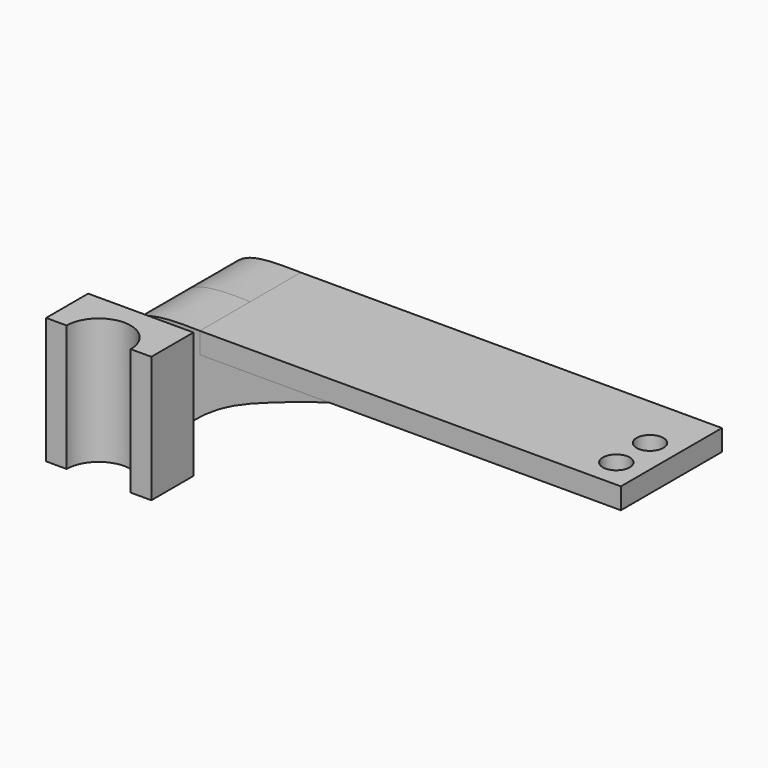
from build123d import *

# Parameters (mm, degrees)
F1_DEPTH      = 19.05
F2_DEPTH      = 19.05
F0_W          = 19.05
F0_H          = 19.05
F3_DEPTH      = 25.4
F3_DEPTH_BACK = 19.05
F4_W          = 31.75
F4_H          = 38.1
F4_W_2        = 19.05
F4_H_2        = 19.05
F5_DEPTH      = 15.875
F7_D          = 19.304
F9_D          = 8.128


with BuildPart() as f1:
    # F0 (on Front) → F1 (new body, symmetric)
    with BuildSketch(Plane.XZ):
        Polygon((73.453836826, -1.6650080707), (-53.546163174, -1.6650080707), (-53.546163174, -8.0150080707), (-14.6733894944, -8.0150080707), (73.453836826, -8.0150080707), align=None)
    extrude(amount=F1_DEPTH, both=True)

    # F9 (through all)
    with Locations(Plane(origin=(0, 0, -8.0150080707), x_dir=(1, 0, 0), z_dir=(0, 0, -1))):
        with Locations((64.970236826, 10.16), (64.970236826, -2.54)):
            Hole(F9_D / 2)


with BuildPart() as f2:
    # F0 (on Front) → F2 (new body, symmetric)
    with BuildSketch(Plane.XZ):
        with BuildLine():
            add(Edge.make_bspline(
                [(-75.771163174, -8.0150080707), (-74.1607508996, -6.1029628681), (-70.2003043439, -1.40071801), (-59.7481949502, -1.5665859823), (-53.546163174, -1.6650080707)],
                knots=[0, 0, 0, 0, 0.4066239127, 1, 1, 1, 1], degree=3))
            Line((-75.771163174, -8.0150080707), (-56.721163174, -8.0150080707))
            Line((-56.721163174, -8.0150080707), (-56.721163174, -27.0650080707))
            add(Edge.make_bspline(
                [(-56.721163174, -27.0650080707), (-53.3356832439, -24.3351180324), (-44.8730943092, -17.5112887062), (-25.9976593517, -11.5759185238), (-14.6733894944, -8.0150080707)],
                knots=[0, 0, 0, 0, 0.4000525083, 1, 1, 1, 1], degree=3))
            Line((-14.6733894944, -8.0150080707), (-53.546163174, -8.0150080707))
            Line((-53.546163174, -8.0150080707), (-53.546163174, -1.6650080707))
        make_face()
    extrude(amount=F2_DEPTH, both=True)


with BuildPart() as f3:
    # F0 (on Front) → F3 (new body, two sides)
    with BuildSketch(Plane.XZ) as f3_sk:
        with Locations((-66.246163174, -17.5400080707)):
            Rectangle(F0_W, F0_H)
    extrude(amount=F3_DEPTH)
    extrude(f3_sk.sketch, amount=-F3_DEPTH_BACK)


with BuildPart() as f5:
    # F4 (on face) → F5 (new body)
    with BuildSketch(Plane.XZ.offset(25.4)):
        with Locations((-66.246163174, -17.5400080707)):
            Rectangle(F4_W, F4_H)
        with Locations((-66.246163174, -17.5400080707)):
            Rectangle(F4_W_2, F4_H_2, mode=Mode.SUBTRACT)
        with Locations((-66.246163174, -17.5400080707)):
            Rectangle(F4_W_2, F4_H_2)
    extrude(amount=F5_DEPTH)

    # F7 (through all)
    with Locations(Plane.XY.offset(1.5099919293)):
        with Locations((-66.246163174, -41.275)):
            Hole(F7_D / 2)


solid = Compound([f1.part, f2.part, f3.part, f5.part])
